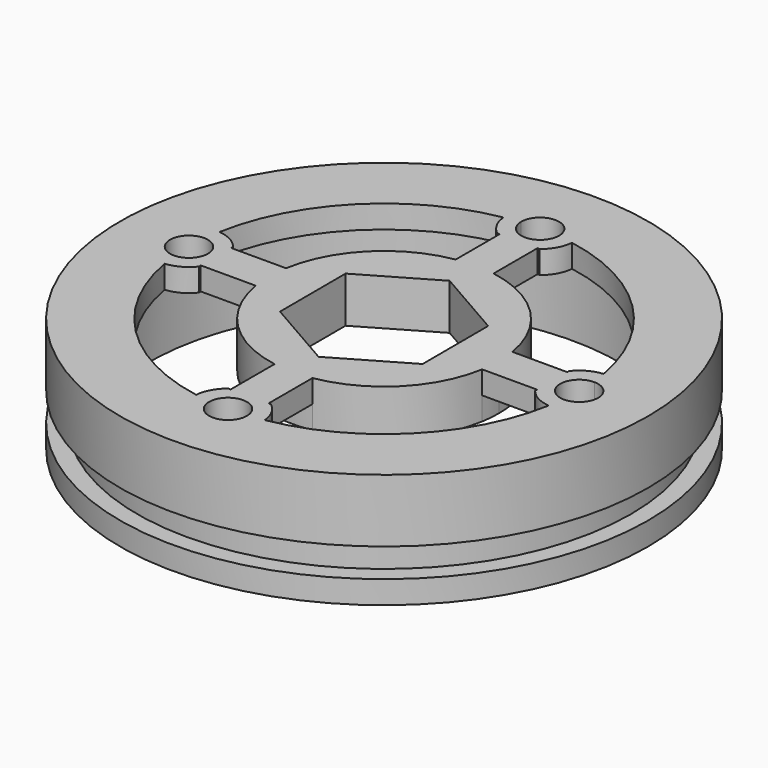
from build123d import *

# Parameters (mm, degrees)
F2_R     = 1.65
F3_DEPTH = 10.001
F5_DEPTH = 2
F7_DEPTH = 10.001
F9_DEPTH = 2


# Not quite as in the source:
# - ends of sketch curves that miss each other by under 0.0002 mm in the source are joined


with BuildPart() as f1:
    # F0 (on Front) → F1 (revolve)
    with BuildSketch(Plane.XZ):
        Polygon((20.5, 16.3456536829), (20.5, 8.3456536829), (23, 8.3456536829), (23, 10.3456536829), (21.5, 10.3456536829), (21.5, 12.8456536829), (23, 12.8456536829), (23, 18.3456536829), (14.75, 18.3456536829), (14.75, 16.3456536829), align=None)
    revolve(axis=Axis((0, 0, 17.3456536829), (0, 0, -1)))

    # F2 (on face) → F3 (cut, through all)
    with BuildSketch(Plane.XY.offset(18.3456536829)):
        with Locations((0, 17)):
            Circle(F2_R)
        with Locations((17, 0)):
            Circle(F2_R)
        with Locations((-17, 0)):
            Circle(F2_R)
        with Locations((0, -17)):
            Circle(F2_R)
    extrude(amount=-F3_DEPTH, mode=Mode.SUBTRACT)

    # F4 (on face) → F5 (join)
    with BuildSketch(Plane.XY.offset(18.3456536829)):
        with BuildLine():
            Line((-1.6499559837, 14.6574262833), (-1.6499626499, 9.8629419168))
            ThreePointArc((-1.6499626499, 9.8629419168), (-7.0714247823, 7.0707108234), (-9.8631084617, 1.6489667897))
            Line((-9.8631084617, 1.6489667897), (-14.6575583453, 1.6487823851))
            ThreePointArc((-14.6575583453, 1.6487823851), (-14.7499999873, -0.0006126499), (-14.6574213285, -1.6499999999))
            Line((-14.6574213285, -1.6499999999), (-9.8629356685, -1.6499999997))
            ThreePointArc((-9.8629356685, -1.6499999997), (-7.0710642548, -7.071071369), (-1.6499900767, -9.8629373285))
            Line((-1.6499900767, -9.8629373285), (-1.6499967429, -14.6574216951))
            ThreePointArc((-1.6499967429, -14.6574216951), (0, -14.75), (1.6499967429, -14.6574216951))
            Line((1.6499967429, -14.6574216951), (1.6499900767, -9.8629373285))
            ThreePointArc((1.6499900767, -9.8629373285), (7.071064255, -7.0710713687), (9.8629356686, -1.649999999))
            Line((9.8629356686, -1.649999999), (14.6574213286, -1.6499999989))
            ThreePointArc((14.6574213286, -1.6499999989), (14.7268371451, -0.8262975866), (14.75, 0))
            ThreePointArc((14.75, 0), (14.7268396846, 0.8262523244), (14.6574314707, 1.6499099011))
            Line((14.6574314707, 1.6499099011), (9.862981587, 1.6497254965))
            ThreePointArc((9.862981587, 1.6497254965), (7.0711528227, 7.0709828), (1.6499626499, 9.8629419168))
            Line((1.6499626499, 9.8629419168), (1.6499559837, 14.6574262833))
            ThreePointArc((1.6499559837, 14.6574262833), (0, 14.75), (-1.6499559837, 14.6574262833))
        make_face()
        with BuildLine():
            Line((-1.649952744, 16.9875123006), (-1.6499559837, 14.6574262833))
            ThreePointArc((-1.6499559837, 14.6574262833), (0, 14.75), (1.6499559837, 14.6574262833))
            Line((1.6499559837, 14.6574262833), (1.649952744, 16.9875123006))
            ThreePointArc((1.649952744, 16.9875123006), (0, 15.35), (-1.649952744, 16.9875123006))
        make_face()
        with BuildLine():
            Line((16.9999365375, 1.6499999988), (14.6574314707, 1.6499099011))
            ThreePointArc((14.6574314707, 1.6499099011), (14.7268396846, 0.8262523244), (14.75, 0))
            ThreePointArc((14.75, 0), (14.7268371451, -0.8262975866), (14.6574213286, -1.6499999989))
            Line((14.6574213286, -1.6499999989), (16.9999365375, -1.6499999988))
            ThreePointArc((16.9999365375, -1.6499999988), (15.35, 0), (16.9999365375, 1.6499999988))
        make_face()
        with BuildLine():
            ThreePointArc((-14.6574213285, -1.6499999999), (-14.7499999873, -0.0006126499), (-14.6575583453, 1.6487823851))
            Line((-14.6575583453, 1.6487823851), (-16.9343843655, 1.6486948136))
            ThreePointArc((-16.9343843655, 1.6486948136), (-15.8103013413, 1.1432922205), (-15.35, 0))
            ThreePointArc((-15.35, 0), (-15.833273811, -1.166726189), (-17, -1.65))
            Line((-17, -1.65), (-14.6574213285, -1.6499999999))
        make_face()
        with BuildLine():
            ThreePointArc((1.6499967429, -14.6574216951), (0, -14.75), (-1.6499967429, -14.6574216951))
            Line((-1.6499967429, -14.6574216951), (-1.65, -16.9999977059))
            ThreePointArc((-1.65, -16.9999977059), (1.1471e-06, -15.35), (1.65, -17))
            Line((1.65, -17), (1.6499967429, -14.6574216951))
        make_face()
    extrude(amount=-F5_DEPTH)

    # F6 (on face) → F7 (cut, through all)
    with BuildSketch(Plane.XY.offset(18.3456536829)):
        with BuildLine():
            ThreePointArc((-1.8447082725, 14.6341911765), (-2.634985421, 15.5658271264), (-2.9882989803, 16.7352941176))
            ThreePointArc((-2.9882989803, 16.7352941176), (-12.0208152802, 12.0208152802), (-16.7352941176, 2.9882989803))
            ThreePointArc((-16.7352941176, 2.9882989803), (-15.5658271264, 2.634985421), (-14.6341911765, 1.8447082725))
            ThreePointArc((-14.6341911765, 1.8447082725), (-10.4298250225, 10.4298250225), (-1.8447082725, 14.6341911765))
        make_face()
        with BuildLine():
            ThreePointArc((2.9882989803, 16.7352941176), (2.634985421, 15.5658271264), (1.8447082725, 14.6341911765))
            ThreePointArc((1.8447082725, 14.6341911765), (10.4298250225, 10.4298250225), (14.6341911765, 1.8447082725))
            ThreePointArc((14.6341911765, 1.8447082725), (15.5658271264, 2.634985421), (16.7352941176, 2.9882989803))
            ThreePointArc((16.7352941176, 2.9882989803), (12.0208152802, 12.0208152802), (2.9882989803, 16.7352941176))
        make_face()
        with BuildLine():
            ThreePointArc((16.7352941176, -2.9882989803), (15.5658271264, -2.634985421), (14.6341911765, -1.8447082725))
            ThreePointArc((14.6341911765, -1.8447082725), (10.4298250225, -10.4298250225), (1.8447082725, -14.6341911765))
            ThreePointArc((1.8447082725, -14.6341911765), (2.634985421, -15.5658271264), (2.9882989803, -16.7352941176))
            ThreePointArc((2.9882989803, -16.7352941176), (12.0208152802, -12.0208152802), (16.7352941176, -2.9882989803))
        make_face()
        with BuildLine():
            ThreePointArc((-1.8447082725, -14.6341911765), (-10.4298250225, -10.4298250225), (-14.6341911765, -1.8447082725))
            ThreePointArc((-14.6341911765, -1.8447082725), (-15.5658271264, -2.634985421), (-16.7352941176, -2.9882989803))
            ThreePointArc((-16.7352941176, -2.9882989803), (-12.0208152802, -12.0208152802), (-2.9882989803, -16.7352941176))
            ThreePointArc((-2.9882989803, -16.7352941176), (-2.634985421, -15.5658271264), (-1.8447082725, -14.6341911765))
        make_face()
        Polygon((0.0182914075, -7.1591199709), (6.2091254673, -3.5637191619), (6.1908340598, 3.595400809), (-0.0182914075, 7.1591199709), (-6.2091254673, 3.5637191619), (-6.1908340598, -3.595400809), align=None)
    extrude(amount=-F7_DEPTH, mode=Mode.SUBTRACT)

    # F8 (on face) → F9 (join)
    with BuildSketch(Plane(origin=(0, 0, 16.3456536829), x_dir=(1, 0, 0), z_dir=(0, 0, -1))):
        with BuildLine():
            ThreePointArc((9.862981587, -1.6497254965), (9.965686526, -0.8277028844), (10, 0))
            ThreePointArc((10, 0), (9.9656750069, 0.8278415651), (9.8629356686, 1.649999999))
            ThreePointArc((9.8629356686, 1.649999999), (7.071064255, 7.0710713687), (1.6499900767, 9.8629373285))
            ThreePointArc((1.6499900767, 9.8629373285), (0, 10), (-1.6499900767, 9.8629373285))
            ThreePointArc((-1.6499900767, 9.8629373285), (-7.0710642548, 7.071071369), (-9.8629356685, 1.6499999997))
            ThreePointArc((-9.8629356685, 1.6499999997), (-9.9999999863, 0.0005237796), (-9.8631084617, -1.6489667897))
            ThreePointArc((-9.8631084617, -1.6489667897), (-7.0714247823, -7.0707108234), (-1.6499626499, -9.8629419168))
            ThreePointArc((-1.6499626499, -9.8629419168), (0, -10), (1.6499626499, -9.8629419168))
            ThreePointArc((1.6499626499, -9.8629419168), (7.0711528227, -7.0709828), (9.862981587, -1.6497254965))
        make_face()
        Polygon((-6.1908340598, 3.595400809), (0.0182914075, 7.1591199709), (6.2091254673, 3.5637191619), (6.1908340598, -3.595400809), (-0.0182914075, -7.1591199709), (-6.2091254673, -3.5637191619), align=None, mode=Mode.SUBTRACT)
    extrude(amount=F9_DEPTH)


solid = f1.part
